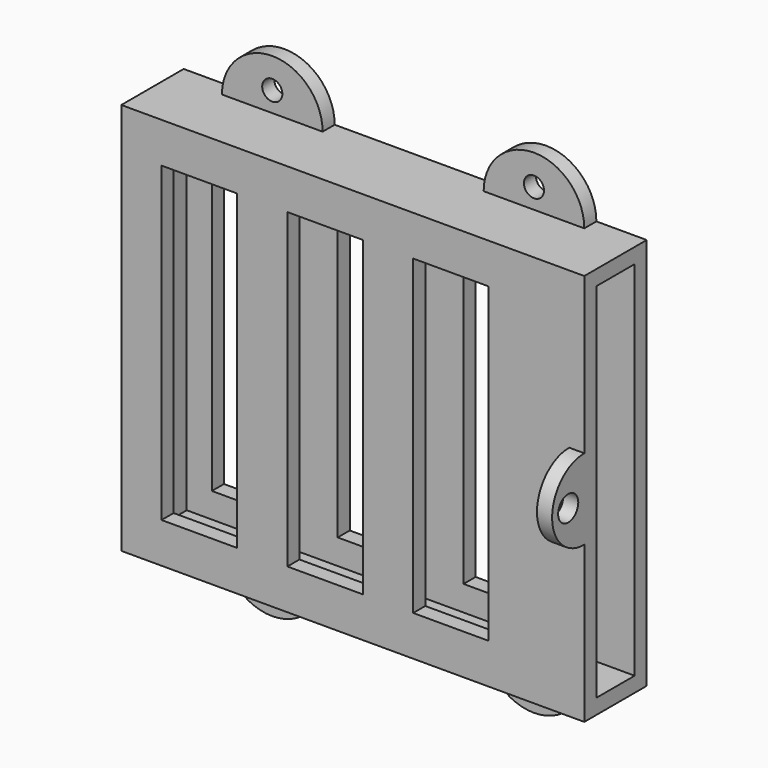
from build123d import *

# Parameters (mm, degrees)
F0_W      = 92
F0_H      = 78
F1_DEPTH  = 15.5
F2_T      = -3
F4_DEPTH  = 3
F5_R      = 2
F6_DEPTH  = 25
F7_W      = 15
F7_H      = 62
F8_DEPTH  = 25
F10_DEPTH = 3
F11_R     = 2.5
F12_DEPTH = 5


# Not quite as in the source:
# - a feature names something its author has since deleted; it is built from what else it names


with BuildPart() as f1:
    # F0 (on Front) → F1 (new body)
    with BuildSketch(Plane.XZ):
        with Locations((-46, 39)):
            Rectangle(F0_W, F0_H)
    extrude(amount=F1_DEPTH)

    # F2
    f2_openings = [f1.faces().sort_by_distance(p)[0] for p in [
        (0, -7.75, 39),
    ]]
    offset(amount=F2_T, openings=f2_openings)

    # F3 (on face) → F4 (join)
    with BuildSketch(Plane(origin=(0, 0, 0), x_dir=(-1, 0, 0), z_dir=(0, 1, 0))):
        with BuildLine():
            Line((62, 78), (82, 78))
            ThreePointArc((82, 78), (72, 88), (62, 78))
        make_face()
        with BuildLine():
            ThreePointArc((62, 0), (72, -10), (82, 0))
            Line((82, 0), (62, 0))
        make_face()
        with BuildLine():
            Line((10, 78), (30, 78))
            ThreePointArc((30, 78), (20, 88), (10, 78))
        make_face()
        with BuildLine():
            ThreePointArc((10, 0), (20, -10), (30, 0))
            Line((30, 0), (10, 0))
        make_face()
    extrude(amount=-F4_DEPTH)

    # F5 (on face) → F6 (cut)
    with BuildSketch(Plane.XZ.offset(3)):
        with Locations((-72, 82)):
            Circle(F5_R)
        with Locations((-72, -4)):
            Circle(F5_R)
        with Locations((-20, 82)):
            Circle(F5_R)
        with Locations((-20, -4)):
            Circle(F5_R)
    extrude(amount=-F6_DEPTH, mode=Mode.SUBTRACT)

    # F7 (on face) → F8 (cut)
    with BuildSketch(Plane.XZ.offset(15.5)):
        with Locations((-76.5, 39)):
            Rectangle(F7_W, F7_H)
        with Locations((-51.5, 39)):
            Rectangle(F7_W, F7_H)
        with Locations((-26.5, 39)):
            Rectangle(F7_W, F7_H)
    extrude(amount=-F8_DEPTH, mode=Mode.SUBTRACT)

    # F9 (on face) → F10 (join)
    with BuildSketch(Plane.YZ):
        with BuildLine():
            Line((-15.5, 31), (-15.5, 47))
            ThreePointArc((-15.5, 47), (-23.5, 39), (-15.5, 31))
        make_face()
    extrude(amount=-F10_DEPTH)

    # F11 (on face) → F12 (cut)
    with BuildSketch(Plane.YZ):
        with Locations((-19.5, 39)):
            Circle(F11_R)
    extrude(amount=-F12_DEPTH, mode=Mode.SUBTRACT)


solid = f1.part
